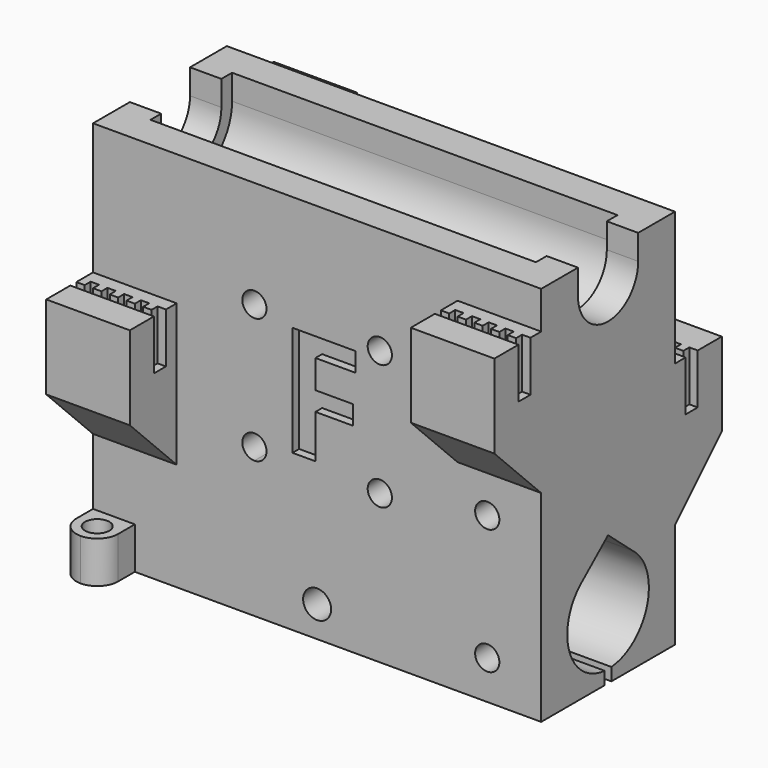
from build123d import *

# Parameters (mm, degrees)
F1_W          = 53.6
F1_H          = 20
F2_DEPTH      = 50.6
F3_W          = 20
F3_H          = 5
F4_DEPTH      = 53.601
F6_DEPTH      = 53.601
F7_DEPTH      = 49.85
F8_DEPTH      = 24.95
F9_DEPTH      = 25.05
F10_DEPTH     = 3.75
F11_W         = 10
F11_H         = 20
F12_DEPTH     = 7
F13_T4_DEPTH  = 61.4336597593
F13_T9_DEPTH  = 61.4336597593
F15_DEPTH     = 6
F17_DEPTH     = 6
F18_W         = 10
F18_H         = 20
F19_DEPTH     = 7
F21_DEPTH     = 6
F23_DEPTH     = 6
F24_T4_DEPTH  = 61.4336597593
F24_T9_DEPTH  = 61.4336597593
F25_R         = 1.45
F25_R_2       = 1.675
F26_DEPTH     = 27.001
F27_R         = 1.45
F28_DEPTH     = 5
F29_TEXT_SIZE = 18.4411155982
F30_DEPTH     = 1
F31_W         = 5
F31_H         = 5
F32_DEPTH     = 5
F34_DEPTH     = 25
F35_R         = 2.49999


# Not quite as in the source:
# - a fillet or chamfer that OpenCascade refuses, or shapes differently, is made with other operations: its cross-section is extruded or revolved along the edge and cut away or added
# - a fillet or chamfer is up to 0.001 mm smaller than in the source, because OpenCascade refuses the exact size
# - a feature names something its author has since deleted; it is built from what else it names
# - Text() gives the source's letters only with a copy of the font that has no kerning and outlines rounded to 1/6400 em; it was checked with that copy


with BuildPart() as f2:
    # F1 (on Top) → F2 (new body)
    with BuildSketch(Plane.XY):
        with Locations((26.8, 10)):
            Rectangle(F1_W, F1_H)
    extrude(amount=F2_DEPTH)

    # F3 (on face) → F4 (cut, through all)
    with BuildSketch(Plane(origin=(0, 0, 0), x_dir=(0, -1, 0), z_dir=(-1, 0, 0))):
        with Locations((-10, 48.1)):
            Rectangle(F3_W, F3_H)
    extrude(amount=-F4_DEPTH, mode=Mode.SUBTRACT)

    # F5 (on face) → F6 (cut, through all)
    with BuildSketch(Plane(origin=(0, 0, 0), x_dir=(0, -1, 0), z_dir=(-1, 0, 0))):
        with BuildLine():
            ThreePointArc((-9.5, 1.5205263386), (-5.5133531452, 3.467204336), (-3.9, 7.6))
            ThreePointArc((-3.9, 7.6), (-4.5568930935, 10.3536497969), (-6.3860941653, 12.5142328616))
            ThreePointArc((-6.3860941653, 12.5142328616), (-8.0982666401, 13.3959822488), (-10, 13.7))
            ThreePointArc((-10, 13.7), (-11.9017333599, 13.3959822488), (-13.6139058347, 12.5142328616))
            ThreePointArc((-13.6139058347, 12.5142328616), (-15.8691099055, 5.937607472), (-10.5, 1.5205263386))
            Line((-10.5, 1.5205263386), (-9.5, 1.5205263386))
        make_face()
        with BuildLine():
            ThreePointArc((-10, 13.7), (-8.0982666401, 13.3959822488), (-6.3860941653, 12.5142328616))
            Line((-6.3860941653, 12.5142328616), (-10, 15.5999502167))
            Line((-10, 15.5999502167), (-10, 13.7))
        make_face()
        with BuildLine():
            Line((-9.5, 0), (-9.5, 1.5205263386))
            ThreePointArc((-9.5, 1.5205263386), (-10, 1.5), (-10.5, 1.5205263386))
            Line((-10.5, 1.5205263386), (-10.5, 0))
            Line((-10.5, 0), (-10, 0))
            Line((-10, 0), (-9.5, 0))
        make_face()
        with BuildLine():
            ThreePointArc((-10.5, 1.5205263386), (-10, 1.5), (-9.5, 1.5205263386))
            Line((-9.5, 1.5205263386), (-10.5, 1.5205263386))
        make_face()
        with BuildLine():
            ThreePointArc((-13.6139058347, 12.5142328616), (-11.9017333599, 13.3959822488), (-10, 13.7))
            Line((-10, 13.7), (-10, 15.5999502167))
            Line((-10, 15.5999502167), (-13.6139058347, 12.5142328616))
        make_face()
        with BuildLine():
            Line((-5.5, 42.6), (-5.5, 45.6))
            Line((-5.5, 45.6), (-6.6458980338, 45.6))
            ThreePointArc((-6.6458980338, 45.6), (-5.7962243847, 44.205699404), (-5.5, 42.6))
        make_face()
        with BuildLine():
            Line((-13.3541019662, 45.6), (-14.5, 45.6))
            Line((-14.5, 45.6), (-14.5, 42.6))
            ThreePointArc((-14.5, 42.6), (-14.2037756153, 44.205699404), (-13.3541019662, 45.6))
        make_face()
        with BuildLine():
            ThreePointArc((-14.5, 42.6), (-10, 38.1), (-5.5, 42.6))
            ThreePointArc((-5.5, 42.6), (-5.7962243847, 44.205699404), (-6.6458980338, 45.6))
            Line((-6.6458980338, 45.6), (-13.3541019662, 45.6))
            ThreePointArc((-13.3541019662, 45.6), (-14.2037756153, 44.205699404), (-14.5, 42.6))
        make_face()
    extrude(amount=-F6_DEPTH, mode=Mode.SUBTRACT)

    # F5 (on face) → F7 (cut)
    with BuildSketch(Plane(origin=(0, 0, 0), x_dir=(0, -1, 0), z_dir=(-1, 0, 0))):
        with BuildLine():
            ThreePointArc((-10.5, 1.5205263386), (-10, 1.5), (-9.5, 1.5205263386))
            Line((-9.5, 1.5205263386), (-10.5, 1.5205263386))
        make_face()
        with BuildLine():
            Line((-5.5, 42.6), (-5.5, 45.6))
            Line((-5.5, 45.6), (-6.6458980338, 45.6))
            ThreePointArc((-6.6458980338, 45.6), (-5.7962243847, 44.205699404), (-5.5, 42.6))
        make_face()
        with BuildLine():
            Line((-13.3541019662, 45.6), (-14.5, 45.6))
            Line((-14.5, 45.6), (-14.5, 42.6))
            ThreePointArc((-14.5, 42.6), (-14.2037756153, 44.205699404), (-13.3541019662, 45.6))
        make_face()
        with BuildLine():
            ThreePointArc((-16.1, 42.6), (-10, 36.5), (-3.9, 42.6))
            ThreePointArc((-3.9, 42.6), (-4.1004668401, 44.1509701788), (-4.68869131, 45.6))
            Line((-4.68869131, 45.6), (-5.5, 45.6))
            Line((-5.5, 45.6), (-5.5, 42.6))
            ThreePointArc((-5.5, 42.6), (-10, 38.1), (-14.5, 42.6))
            Line((-14.5, 42.6), (-14.5, 45.6))
            Line((-14.5, 45.6), (-15.31130869, 45.6))
            ThreePointArc((-15.31130869, 45.6), (-15.8995331599, 44.1509701788), (-16.1, 42.6))
        make_face()
        with BuildLine():
            Line((-5.5, 45.6), (-4.68869131, 45.6))
            ThreePointArc((-4.68869131, 45.6), (-10, 48.7), (-15.31130869, 45.6))
            Line((-15.31130869, 45.6), (-14.5, 45.6))
            Line((-14.5, 45.6), (-13.3541019662, 45.6))
            ThreePointArc((-13.3541019662, 45.6), (-10, 47.1), (-6.6458980338, 45.6))
            Line((-6.6458980338, 45.6), (-5.5, 45.6))
        make_face()
        with BuildLine():
            Line((-3.9, 42.6), (-3.9, 45.6))
            Line((-3.9, 45.6), (-4.68869131, 45.6))
            ThreePointArc((-4.68869131, 45.6), (-4.1004668401, 44.1509701788), (-3.9, 42.6))
        make_face()
        with BuildLine():
            Line((-15.31130869, 45.6), (-16.1, 45.6))
            Line((-16.1, 45.6), (-16.1, 42.6))
            ThreePointArc((-16.1, 42.6), (-15.8995331599, 44.1509701788), (-15.31130869, 45.6))
        make_face()
    extrude(amount=-F7_DEPTH, mode=Mode.SUBTRACT)

    # F5 (on face) → F8, piece 2 (join)
    with BuildSketch(Plane(origin=(0, 0, 0), x_dir=(0, -1, 0), z_dir=(-1, 0, 0))):
        with BuildLine():
            ThreePointArc((-16.1, 42.6), (-10, 36.5), (-3.9, 42.6))
            ThreePointArc((-3.9, 42.6), (-4.1004668401, 44.1509701788), (-4.68869131, 45.6))
            Line((-4.68869131, 45.6), (-5.5, 45.6))
            Line((-5.5, 45.6), (-5.5, 42.6))
            ThreePointArc((-5.5, 42.6), (-10, 38.1), (-14.5, 42.6))
            Line((-14.5, 42.6), (-14.5, 45.6))
            Line((-14.5, 45.6), (-15.31130869, 45.6))
            ThreePointArc((-15.31130869, 45.6), (-15.8995331599, 44.1509701788), (-16.1, 42.6))
        make_face()
        with BuildLine():
            Line((-15.31130869, 45.6), (-16.1, 45.6))
            Line((-16.1, 45.6), (-16.1, 42.6))
            ThreePointArc((-16.1, 42.6), (-15.8995331599, 44.1509701788), (-15.31130869, 45.6))
        make_face()
        with BuildLine():
            Line((-3.9, 42.6), (-3.9, 45.6))
            Line((-3.9, 45.6), (-4.68869131, 45.6))
            ThreePointArc((-4.68869131, 45.6), (-4.1004668401, 44.1509701788), (-3.9, 42.6))
        make_face()
    extrude(amount=-F8_DEPTH)


with BuildPart() as f8:
    # F5 (on face) → F8 (new body)
    with BuildSketch(Plane(origin=(0, 0, 0), x_dir=(0, -1, 0), z_dir=(-1, 0, 0))):
        with BuildLine():
            ThreePointArc((-10.5, 1.5205263386), (-10, 1.5), (-9.5, 1.5205263386))
            Line((-9.5, 1.5205263386), (-10.5, 1.5205263386))
        make_face()
    extrude(amount=-F8_DEPTH)


with BuildPart() as f9_tool:
    # F5 (on face) → F9 (new body)
    with BuildSketch(Plane(origin=(0, 0, 0), x_dir=(0, -1, 0), z_dir=(-1, 0, 0))):
        with BuildLine():
            Line((-9.5, 0), (-9.5, 1.5205263386))
            ThreePointArc((-9.5, 1.5205263386), (-10, 1.5), (-10.5, 1.5205263386))
            Line((-10.5, 1.5205263386), (-10.5, 0))
            Line((-10.5, 0), (-10, 0))
            Line((-10, 0), (-9.5, 0))
        make_face()
        with BuildLine():
            ThreePointArc((-10.5, 1.5205263386), (-10, 1.5), (-9.5, 1.5205263386))
            Line((-9.5, 1.5205263386), (-10.5, 1.5205263386))
        make_face()
        with BuildLine():
            ThreePointArc((-10, 13.7), (-8.0982666401, 13.3959822488), (-6.3860941653, 12.5142328616))
            Line((-6.3860941653, 12.5142328616), (-10, 15.5999502167))
            Line((-10, 15.5999502167), (-10, 13.7))
        make_face()
        with BuildLine():
            ThreePointArc((-13.6139058347, 12.5142328616), (-11.9017333599, 13.3959822488), (-10, 13.7))
            Line((-10, 13.7), (-10, 15.5999502167))
            Line((-10, 15.5999502167), (-13.6139058347, 12.5142328616))
        make_face()
        with BuildLine():
            ThreePointArc((-9.5, 1.5205263386), (-5.5133531452, 3.467204336), (-3.9, 7.6))
            ThreePointArc((-3.9, 7.6), (-4.5568930935, 10.3536497969), (-6.3860941653, 12.5142328616))
            ThreePointArc((-6.3860941653, 12.5142328616), (-8.0982666401, 13.3959822488), (-10, 13.7))
            ThreePointArc((-10, 13.7), (-11.9017333599, 13.3959822488), (-13.6139058347, 12.5142328616))
            ThreePointArc((-13.6139058347, 12.5142328616), (-15.8691099055, 5.937607472), (-10.5, 1.5205263386))
            Line((-10.5, 1.5205263386), (-9.5, 1.5205263386))
        make_face()
        with BuildLine():
            ThreePointArc((-16.1, 42.6), (-10, 36.5), (-3.9, 42.6))
            ThreePointArc((-3.9, 42.6), (-4.1004668401, 44.1509701788), (-4.68869131, 45.6))
            Line((-4.68869131, 45.6), (-5.5, 45.6))
            Line((-5.5, 45.6), (-5.5, 42.6))
            ThreePointArc((-5.5, 42.6), (-10, 38.1), (-14.5, 42.6))
            Line((-14.5, 42.6), (-14.5, 45.6))
            Line((-14.5, 45.6), (-15.31130869, 45.6))
            ThreePointArc((-15.31130869, 45.6), (-15.8995331599, 44.1509701788), (-16.1, 42.6))
        make_face()
        with BuildLine():
            Line((-15.31130869, 45.6), (-16.1, 45.6))
            Line((-16.1, 45.6), (-16.1, 42.6))
            ThreePointArc((-16.1, 42.6), (-15.8995331599, 44.1509701788), (-15.31130869, 45.6))
        make_face()
        with BuildLine():
            Line((-3.9, 42.6), (-3.9, 45.6))
            Line((-3.9, 45.6), (-4.68869131, 45.6))
            ThreePointArc((-4.68869131, 45.6), (-4.1004668401, 44.1509701788), (-3.9, 42.6))
        make_face()
    extrude(amount=-F9_DEPTH)


with BuildPart() as f2_1:
    add(f2.part)

    # F9: cut by f9_tool
    add(f9_tool.part, mode=Mode.SUBTRACT)

    # F5 (on face) → F10, piece 2 (join)
    with BuildSketch(Plane(origin=(0, 0, 0), x_dir=(0, -1, 0), z_dir=(-1, 0, 0))):
        with BuildLine():
            ThreePointArc((-16.1, 42.6), (-10, 36.5), (-3.9, 42.6))
            ThreePointArc((-3.9, 42.6), (-4.1004668401, 44.1509701788), (-4.68869131, 45.6))
            Line((-4.68869131, 45.6), (-5.5, 45.6))
            Line((-5.5, 45.6), (-5.5, 42.6))
            ThreePointArc((-5.5, 42.6), (-10, 38.1), (-14.5, 42.6))
            Line((-14.5, 42.6), (-14.5, 45.6))
            Line((-14.5, 45.6), (-15.31130869, 45.6))
            ThreePointArc((-15.31130869, 45.6), (-15.8995331599, 44.1509701788), (-16.1, 42.6))
        make_face()
        with BuildLine():
            Line((-15.31130869, 45.6), (-16.1, 45.6))
            Line((-16.1, 45.6), (-16.1, 42.6))
            ThreePointArc((-16.1, 42.6), (-15.8995331599, 44.1509701788), (-15.31130869, 45.6))
        make_face()
        with BuildLine():
            Line((-3.9, 42.6), (-3.9, 45.6))
            Line((-3.9, 45.6), (-4.68869131, 45.6))
            ThreePointArc((-4.68869131, 45.6), (-4.1004668401, 44.1509701788), (-3.9, 42.6))
        make_face()
    extrude(amount=-F10_DEPTH)

    # F11 (on face) → F12 (join)
    with BuildSketch(Plane.XZ):
        with Locations((5, 19.9)):
            Rectangle(F11_W, F11_H)
        with Locations((48.6, 31.1)):
            Rectangle(F11_W, F11_H)
    extrude(amount=F12_DEPTH)

    # F13: chamfer of 10 on 2 edges, made by hand


with BuildPart() as f8_1:
    add(f8.part)

    # F9: cut by f9_tool
    add(f9_tool.part, mode=Mode.SUBTRACT)


with BuildPart() as f10:
    # F5 (on face) → F10 (new body)
    with BuildSketch(Plane(origin=(0, 0, 0), x_dir=(0, -1, 0), z_dir=(-1, 0, 0))):
        with BuildLine():
            ThreePointArc((-10.5, 1.5205263386), (-10, 1.5), (-9.5, 1.5205263386))
            Line((-9.5, 1.5205263386), (-10.5, 1.5205263386))
        make_face()
    extrude(amount=-F10_DEPTH)


with BuildPart() as f13_tool2:
    # F13_s3 → F13_t4 (new body)
    with BuildSketch(Plane.YZ.offset(-25.7168298797)):
        Polygon((3, 9.9), (-7, 19.9), (-7, 9.9), align=None)
    extrude(amount=F13_T4_DEPTH)

    split(bisect_by=Plane.XZ, keep=Keep.TOP)


with BuildPart() as f2_2:
    add(f2_1.part)

    # F13_t1: cut F13_tool2
    add(f13_tool2.part, mode=Mode.SUBTRACT)


with BuildPart() as f13_tool7:
    # F13_s8 → F13_t9 (new body)
    with BuildSketch(Plane.YZ.offset(17.8831701203)):
        Polygon((3, 21.1), (-7, 31.1), (-7, 21.1), align=None)
    extrude(amount=F13_T9_DEPTH)

    split(bisect_by=Plane.XZ, keep=Keep.TOP)


with BuildPart() as f2_3:
    add(f2_2.part)

    # F13_t6: cut F13_tool7
    add(f13_tool7.part, mode=Mode.SUBTRACT)

    # F14 (on face) → F15 (cut)
    with BuildSketch(Plane.XY.offset(29.9)):
        Polygon((0, -2.5), (0, -3.4), (10, -3.4), (10, -2.5), (10, -1.6), (9, -1.6), (9, -2.5), (8, -2.5), (8, -1.6), (7, -1.6), (7, -2.5), (6, -2.5), (6, -1.6), (5.2958247252, -1.6), (5, -1.6), (5, -2.5), (4, -2.5), (4, -1.6), (3, -1.6), (3, -2.5), (2, -2.5), (2, -1.6), (1, -1.6), (1, -2.5), align=None)
    extrude(amount=-F15_DEPTH, mode=Mode.SUBTRACT)

    # F16 (on face) → F17 (cut)
    with BuildSketch(Plane.XY.offset(41.1)):
        Polygon((43.6, -2.5), (43.6, -3.4), (53.6, -3.4), (53.6, -2.5), (53.6, -1.6), (52.6, -1.6), (52.6, -2.5), (51.6, -2.5), (51.6, -1.6), (50.6, -1.6), (50.6, -2.5), (49.6, -2.5), (49.6, -1.6), (48.8349036932, -1.6), (48.6, -1.6), (48.6, -2.5), (47.6, -2.5), (47.6, -1.6), (46.6, -1.6), (46.6, -2.5), (45.6, -2.5), (45.6, -1.6), (44.6, -1.6), (44.6, -2.5), align=None)
    extrude(amount=-F17_DEPTH, mode=Mode.SUBTRACT)

    # F18 (on face) → F19 (join)
    with BuildSketch(Plane(origin=(0, 20, 0), x_dir=(-1, 0, 0), z_dir=(0, 1, 0))):
        with Locations((-48.6, 19.6)):
            Rectangle(F18_W, F18_H)
        with Locations((-5, 31.1)):
            Rectangle(F18_W, F18_H)
    extrude(amount=F19_DEPTH)

    # F20 (on face) → F21 (cut)
    with BuildSketch(Plane.XY.offset(29.6)):
        Polygon((43.6, 22.5), (43.6, 21.6), (48.6, 21.6), (53.6, 21.6), (53.6, 22.5), (53.6, 23.4), (52.6, 23.4), (52.6, 22.5), (51.6, 22.5), (51.6, 23.4), (50.6, 23.4), (50.6, 22.5), (49.6, 22.5), (49.6, 23.4), (48.6, 23.4), (48.6, 22.5), (47.6, 22.5), (47.6, 23.4), (46.6, 23.4), (46.6, 22.5), (45.6, 22.5), (45.6, 23.4), (44.6, 23.4), (44.6, 22.5), align=None)
    extrude(amount=-F21_DEPTH, mode=Mode.SUBTRACT)

    # F22 (on face) → F23 (cut)
    with BuildSketch(Plane.XY.offset(41.1)):
        Polygon((7, 22.5), (6, 22.5), (6, 23.4), (5, 23.4), (5, 22.5), (4, 22.5), (4, 23.4), (3, 23.4), (3, 22.5), (2, 22.5), (2, 23.4), (1, 23.4), (1, 22.5), (0, 22.5), (0, 21.6), (5, 21.6), (10, 21.6), (10, 22.5), (10, 23.4), (9, 23.4), (9, 22.5), (8, 22.5), (8, 23.4), (7, 23.4), align=None)
    extrude(amount=-F23_DEPTH, mode=Mode.SUBTRACT)

    # F24: chamfer of 10 on 2 edges, made by hand


with BuildPart() as f24_tool2:
    # F24_s3 → F24_t4 (new body)
    with BuildSketch(Plane.YZ.offset(35.7168298797)):
        Polygon((27, 31.1), (17, 21.1), (27, 21.1), align=None)
    extrude(amount=-F24_T4_DEPTH)

    split(bisect_by=Plane.XZ.offset(-20), keep=Keep.BOTTOM)


with BuildPart() as f2_4:
    add(f2_3.part)

    # F24_t1: cut F24_tool2
    add(f24_tool2.part, mode=Mode.SUBTRACT)


with BuildPart() as f24_tool7:
    # F24_s8 → F24_t9 (new body)
    with BuildSketch(Plane.YZ.offset(79.3168298797)):
        Polygon((17, 9.6), (27, 19.6), (27, 9.6), align=None)
    extrude(amount=-F24_T9_DEPTH)

    split(bisect_by=Plane.XZ.offset(-20), keep=Keep.BOTTOM)


with BuildPart() as f2_5:
    add(f2_4.part)

    # F24_t6: cut F24_tool7
    add(f24_tool7.part, mode=Mode.SUBTRACT)

    # F25 (on face) → F26 (cut, through all)
    with BuildSketch(Plane.XZ):
        with BuildLine():
            ThreePointArc((17.85, 32.8), (19.3, 31.35), (20.75, 32.8))
            ThreePointArc((20.75, 32.8), (19.3, 34.25), (17.85, 32.8))
        make_face()
        with BuildLine():
            ThreePointArc((34.3, 34.25), (33.2746951673, 31.7746951673), (35.75, 32.8))
            ThreePointArc((35.75, 32.8), (35.3253048327, 33.8253048327), (34.3, 34.25))
        make_face()
        with BuildLine():
            ThreePointArc((19.3, 16.35), (20.3253048327, 16.7746951673), (20.75, 17.8))
            ThreePointArc((20.75, 17.8), (18.2746951673, 18.8253048327), (19.3, 16.35))
        make_face()
        with Locations((34.3, 17.8)):
            Circle(F25_R)
        with Locations((26.8, 3.675)):
            Circle(F25_R_2)
        with BuildLine():
            ThreePointArc((35.75, 32.8), (35.3253048327, 33.8253048327), (34.3, 34.25))
            ThreePointArc((34.3, 34.25), (33.2746951673, 31.7746951673), (35.75, 32.8))
        make_face()
        with BuildLine():
            ThreePointArc((20.75, 17.8), (18.2746951673, 18.8253048327), (19.3, 16.35))
            ThreePointArc((19.3, 16.35), (20.3253048327, 16.7746951673), (20.75, 17.8))
        make_face()
    extrude(amount=-F26_DEPTH, mode=Mode.SUBTRACT)

    # F27 (on face) → F28 (cut)
    with BuildSketch(Plane.XZ):
        with Locations((47.15, 19.65)):
            Circle(F27_R)
        with Locations((47.15, 4.65)):
            Circle(F27_R)
    extrude(amount=-F28_DEPTH, mode=Mode.SUBTRACT)

    # F29 (on face) → F30 (cut)
    with BuildSketch(Plane.XZ):
        with Locations((22.1983653734, 18.6611983846)):
            Text('F', F29_TEXT_SIZE, font='Open Sans', font_style=FontStyle.BOLD, text_align=(TextAlign.LEFT, TextAlign.BOTTOM))
    extrude(amount=-F30_DEPTH, mode=Mode.SUBTRACT)

    # F31 (on face) → F32 (join)
    with BuildSketch(Plane.XZ):
        with Locations((2.5, 2.5)):
            Rectangle(F31_W, F31_H)
    extrude(amount=F32_DEPTH)

    # F33 (on face) → F34 (cut)
    with BuildSketch(Plane.XY.offset(5)):
        with BuildLine():
            Line((1.05, -2.5), (3.95, -2.5))
            ThreePointArc((3.95, -2.5), (2.5, -1.05), (1.05, -2.5))
        make_face()
        with BuildLine():
            ThreePointArc((1.05, -2.5), (2.5, -3.95), (3.95, -2.5))
            Line((3.95, -2.5), (1.05, -2.5))
        make_face()
    extrude(amount=-F34_DEPTH, mode=Mode.SUBTRACT)

    # F35 (radius 2.5 in the source; OpenCascade refuses exactly that, so slightly less here)
    f35_edges = [f2_5.edges().sort_by_distance(p)[0] for p in [
        (0, -5, 2.5),
        (5, -5, 2.5),
    ]]
    fillet(f35_edges, radius=F35_R)


solid = Compound([f10.part, f2_5.part])
